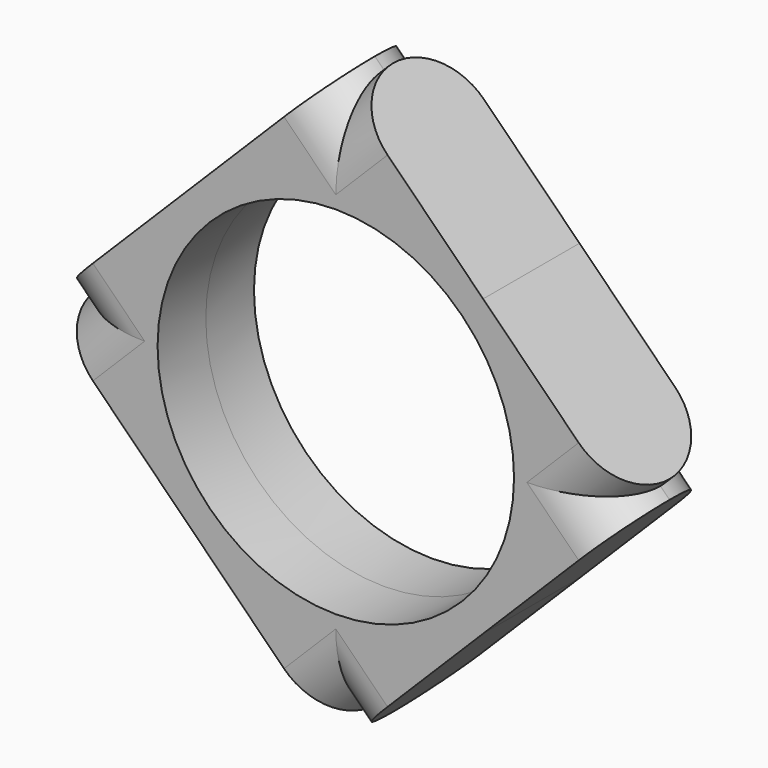
from build123d import *

# Parameters (mm, degrees)
F0_R          = 8.875
F1_DEPTH      = 3
F1_DEPTH_BACK = 3
F2_R          = 2.99999


# Not quite as in the source:
# - a fillet or chamfer is up to 0.001 mm smaller than in the source, because OpenCascade refuses the exact size


with BuildPart() as f1:
    # F0 (on Front) → F1 (new body, two sides)
    with BuildSketch(Plane.XZ) as f1_sk:
        with BuildLine():
            ThreePointArc((-7.3362328356, 7.3362328741), (1.36e-08, 10.375), (7.3362328548, 7.3362328548))
            Line((7.3362328548, 7.3362328548), (0.4560838739, 14.2163818358))
            Line((0.4560838739, 14.2163818358), (0, 13.7602979619))
            Line((0, 13.7602979619), (-0.4560838739, 14.2163818358))
            Line((-0.4560838739, 14.2163818358), (-7.3362328356, 7.3362328741))
        make_face()
        with BuildLine():
            ThreePointArc((-7.3362328073, -7.3362329024), (-10.375, -2e-08), (-7.3362328356, 7.3362328741))
            Line((-7.3362328356, 7.3362328741), (-14.2163818358, 0.4560838739))
            Line((-14.2163818358, 0.4560838739), (-13.7602979619, 0))
            Line((-13.7602979619, 0), (-14.2163818358, -0.4560838739))
            Line((-14.2163818358, -0.4560838739), (-7.3362328073, -7.3362329024))
        make_face()
        with BuildLine():
            ThreePointArc((7.3362328617, -7.3362328479), (9.5852501517, -3.9703406063), (10.375, 0))
            ThreePointArc((10.375, 0), (9.5852501498, 3.9703406108), (7.3362328548, 7.3362328548))
            ThreePointArc((7.3362328548, 7.3362328548), (1.36e-08, 10.375), (-7.3362328356, 7.3362328741))
            ThreePointArc((-7.3362328356, 7.3362328741), (-10.375, -2e-08), (-7.3362328073, -7.3362329024))
            ThreePointArc((-7.3362328073, -7.3362329024), (3.85e-08, -10.375), (7.3362328617, -7.3362328479))
        make_face()
        Circle(F0_R, mode=Mode.SUBTRACT)
        with BuildLine():
            ThreePointArc((7.3362328548, 7.3362328548), (9.5852501498, 3.9703406108), (10.375, 0))
            ThreePointArc((10.375, 0), (9.5852501517, -3.9703406063), (7.3362328617, -7.3362328479))
            Line((7.3362328617, -7.3362328479), (14.2163818358, -0.4560838739))
            Line((14.2163818358, -0.4560838739), (13.7602979619, 0))
            Line((13.7602979619, 0), (14.2163818358, 0.4560838739))
            Line((14.2163818358, 0.4560838739), (7.3362328548, 7.3362328548))
        make_face()
        with BuildLine():
            Line((0.4560838739, -14.2163818358), (7.3362328617, -7.3362328479))
            ThreePointArc((7.3362328617, -7.3362328479), (3.85e-08, -10.375), (-7.3362328073, -7.3362329024))
            Line((-7.3362328073, -7.3362329024), (-0.4560838739, -14.2163818358))
            Line((-0.4560838739, -14.2163818358), (0, -13.7602979619))
            Line((0, -13.7602979619), (0.4560838739, -14.2163818358))
        make_face()
    extrude(amount=F1_DEPTH)
    extrude(f1_sk.sketch, amount=-F1_DEPTH_BACK)

    # F2 (radius 3 in the source; OpenCascade refuses exactly that, so slightly less here)
    f2_edges = [f1.edges().sort_by_distance(p)[0] for p in [
        (0.228042, -3, 13.98834),
        (-0.228042, -3, 13.98834),
        (13.98834, -3, 0.228042),
        (13.98834, -3, -0.228042),
        (0.228042, -3, -13.98834),
        (-0.228042, -3, -13.98834),
        (-13.98834, -3, 0.228042),
        (-13.98834, -3, -0.228042),
        (-13.98834, 3, 0.228042),
        (-13.98834, 3, -0.228042),
        (-0.228042, 3, -13.98834),
        (0.228042, 3, -13.98834),
        (13.98834, 3, 0.228042),
        (13.98834, 3, -0.228042),
        (0.228042, 3, 13.98834),
        (-0.228042, 3, 13.98834),
    ]]
    fillet(f2_edges, radius=F2_R)


solid = f1.part
